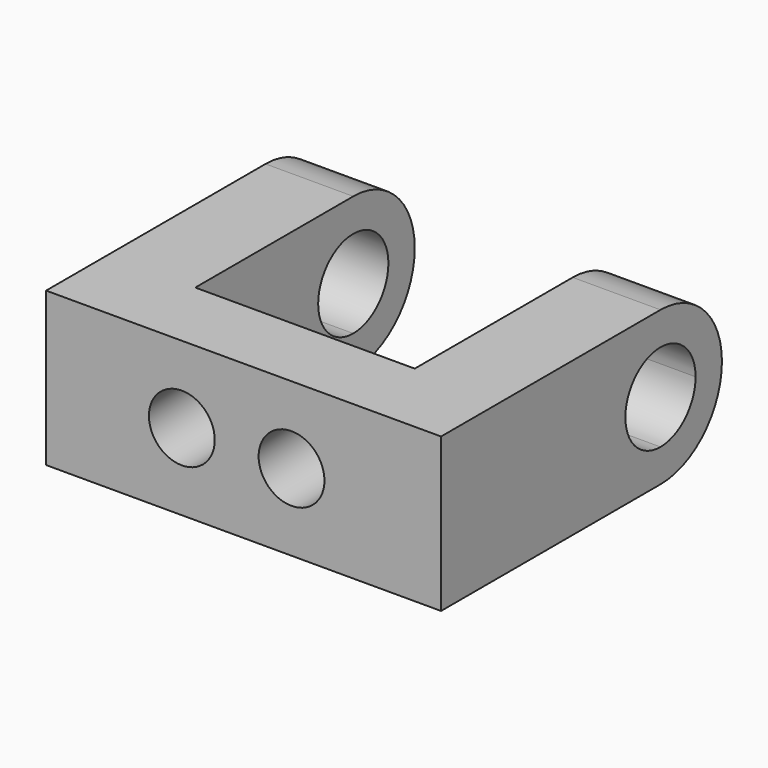
from build123d import *
from build123d import SkipClean  # not in build123d's __all__

# Parameters (mm, degrees)
F1_DEPTH = 7
F3_DEPTH = 18
F4_DEPTH = 4
F6_DEPTH = 4
F7_R     = 1.5
F8_DEPTH = 3.5


with BuildPart() as f1:
    # F0 (on Top) → F1 (new body)
    with BuildSketch(Plane.XY):
        Polygon((-8.6863613641, -3.3171127737), (0.3136386359, -3.3171127737), (9.3136386359, -3.3171127737), (9.3136386359, 0.1828872263), (9.3136386359, 9.1828872263), (5.3136386359, 9.1828872263), (5.3136386359, 0.1828872263), (-4.6863613641, 0.1828872263), (-4.6863613641, 9.1828872263), (-8.6863613641, 9.1828872263), (-8.6863613641, 0.1828872263), align=None)
    extrude(amount=F1_DEPTH)

    # F2 (on face) → F3 (cut, through all)
    with BuildSketch(Plane(origin=(-8.6863613641, 0, 0), x_dir=(0, -1, 0), z_dir=(-1, 0, 0))):
        with BuildLine():
            Line((-9.1828872263, 5.5), (-9.1828872263, 1.5))
            ThreePointArc((-9.1828872263, 1.5), (-7.768673664, 2.0857864376), (-7.1828872263, 3.5))
            ThreePointArc((-7.1828872263, 3.5), (-7.768673664, 4.9142135624), (-9.1828872263, 5.5))
        make_face()
    extrude(amount=-F3_DEPTH, mode=Mode.SUBTRACT)

    # F2 (on face) → F4 (join, through all)
    with BuildSketch(Plane(origin=(-8.6863613641, 0, 0), x_dir=(0, -1, 0), z_dir=(-1, 0, 0))):
        with BuildLine():
            ThreePointArc((-9.1828872263, 7), (-12.6828872263, 3.5), (-9.1828872263, 0))
            Line((-9.1828872263, 0), (-9.1828872263, 1.5))
            ThreePointArc((-9.1828872263, 1.5), (-11.1828872263, 3.5), (-9.1828872263, 5.5))
            Line((-9.1828872263, 5.5), (-9.1828872263, 7))
        make_face()
    with SkipClean():  # cleaning this boolean's faces spoils the solid; the shape is the same uncleaned
        extrude(amount=-F4_DEPTH)

    # F5 (on face) → F6 (join, through all)
    with BuildSketch(Plane.YZ.offset(9.3136386359)):
        with BuildLine():
            ThreePointArc((9.1828872263, 1.5), (7.1828872263, 3.5), (9.1828872263, 5.5))
            Line((9.1828872263, 5.5), (9.1828872263, 7))
            ThreePointArc((9.1828872263, 7), (5.6828872263, 3.5), (9.1828872263, 0))
            Line((9.1828872263, 0), (9.1828872263, 1.5))
        make_face()
        with BuildLine():
            Line((9.1828872263, 7), (9.1828872263, 5.5))
            ThreePointArc((9.1828872263, 5.5), (10.5971007887, 4.9142135624), (11.1828872263, 3.5))
            ThreePointArc((11.1828872263, 3.5), (10.5971007887, 2.0857864376), (9.1828872263, 1.5))
            Line((9.1828872263, 1.5), (9.1828872263, 0))
            ThreePointArc((9.1828872263, 0), (11.6577609605, 1.0251262658), (12.6828872263, 3.5))
            ThreePointArc((12.6828872263, 3.5), (11.6577609605, 5.9748737342), (9.1828872263, 7))
        make_face()
        with BuildLine():
            ThreePointArc((9.1828872263, 0), (5.6828872263, 3.5), (9.1828872263, 7))
            Line((9.1828872263, 7), (-3.3171127737, 7))
            Line((-3.3171127737, 7), (-3.3171127737, 0))
            Line((-3.3171127737, 0), (9.1828872263, 0))
        make_face()
    extrude(amount=-F6_DEPTH)

    # F7 (on face) → F8 (cut, through all)
    with BuildSketch(Plane.XZ.offset(3.3171127737)):
        with Locations((-2.5, 3.5)):
            Circle(F7_R)
        with Locations((2.5, 3.5)):
            Circle(F7_R)
    extrude(amount=-F8_DEPTH, mode=Mode.SUBTRACT)


solid = f1.part
